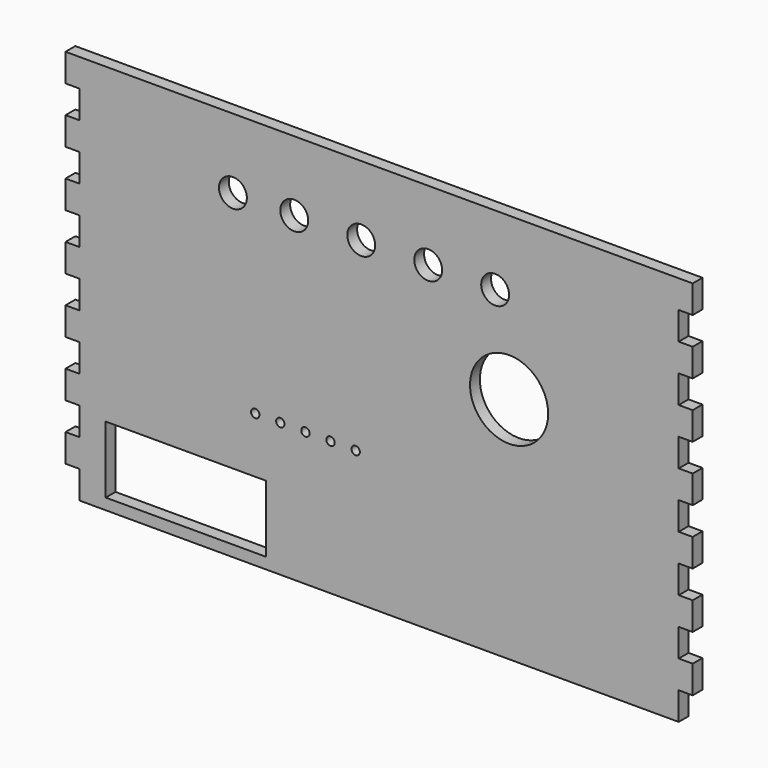
from build123d import *

# Parameters (mm, degrees)
F0_W      = 285.496
F0_H      = 177.8
F1_DEPTH  = 5.588
F2_W      = 73.025
F2_H      = 30.48
F3_DEPTH  = 25.4
F5_D      = 12.7
F7_D      = 12.7
F9_D      = 3.81
F10_W     = 6.35
F10_H     = 12.7
F11_DEPTH = 25.4
F12_R     = 17.78
F13_DEPTH = 25.4


# Not quite as in the source:
# - a pattern or mirror of a feature is missing from the dataset's text; its kind, count and spacing are read off the source's solid


with BuildPart() as f1:
    # F0 (on Front) → F1 (new body)
    with BuildSketch(Plane.XZ):
        Rectangle(F0_W, F0_H)
    extrude(amount=F1_DEPTH)

    # F2 (on Front) → F3 (cut)
    with BuildSketch(Plane.XZ):
        with Locations((-87.9475, -68.58)):
            Rectangle(F2_W, F2_H)
    extrude(amount=F3_DEPTH, mode=Mode.SUBTRACT)

    # F5 (through all)
    with Locations(Plane(origin=(0, 0, 0), x_dir=(1, 0, 0), z_dir=(0, 1, 0))):
        with Locations((-66.548, -57.15)):
            Hole(F5_D / 2)

    # F7 (through all)
    with Locations(Plane(origin=(0, 0, 0), x_dir=(1, 0, 0), z_dir=(0, 1, 0))):
        with Locations((-38.608, -57.15), (-8.128, -57.15), (22.352, -57.15), (52.832, -57.15)):
            Hole(F7_D / 2)

    # F9 (through all)
    with Locations(Plane(origin=(0, 0, 0), x_dir=(1, 0, 0), z_dir=(0, 1, 0))):
        with Locations((-56.388, 27.94), (-44.958, 27.94), (-33.528, 27.94), (-22.098, 27.94), (-10.668, 27.94)):
            Hole(F9_D / 2)

    # F10 (on Front) → F11 (cut)
    with BuildSketch(Plane.XZ):
        with Locations((139.573, 69.85)):
            Rectangle(F10_W, F10_H)
        with Locations((139.573, 19.05)):
            Rectangle(F10_W, F10_H)
        with Locations((139.573, -6.35)):
            Rectangle(F10_W, F10_H)
        with Locations((139.573, -31.75)):
            Rectangle(F10_W, F10_H)
        with Locations((139.573, -57.15)):
            Rectangle(F10_W, F10_H)
        with Locations((139.573, -82.55)):
            Rectangle(F10_W, F10_H)
        with Locations((139.573, 44.45)):
            Rectangle(F10_W, F10_H)
    f11 = extrude(amount=F11_DEPTH, mode=Mode.SUBTRACT)

    # F11_copies: F11 across plane
    add(f11.mirror(Plane(origin=(0, 0, 0), x_dir=(0, 0, -1), z_dir=(-1, 0, 0))), mode=Mode.SUBTRACT)

    # F12 (on Front) → F13 (cut)
    with BuildSketch(Plane.XZ):
        with Locations((59.182, 15.24)):
            Circle(F12_R)
    extrude(amount=F13_DEPTH, mode=Mode.SUBTRACT)


solid = f1.part
